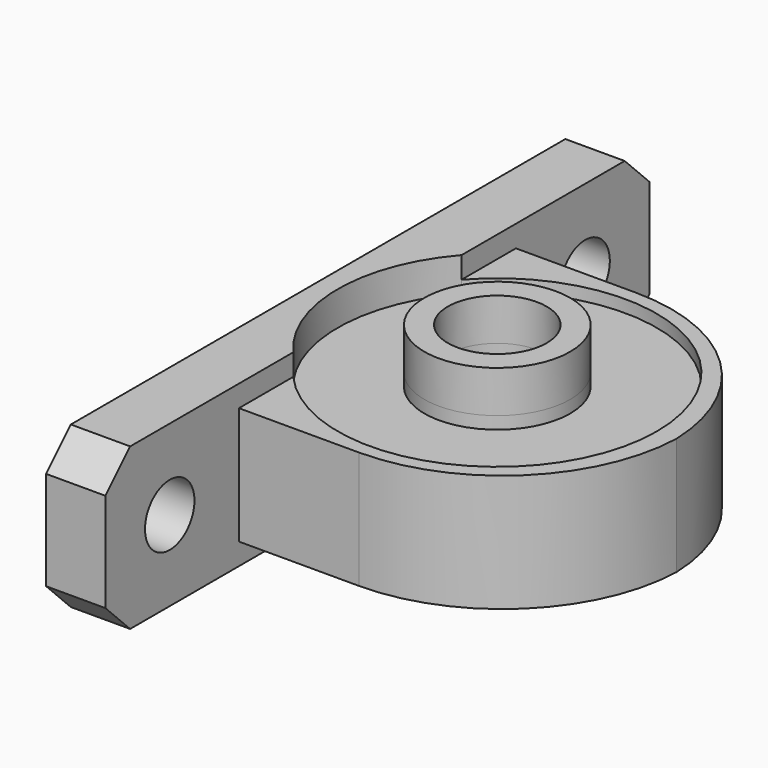
from build123d import *

# Parameters (mm, degrees)
F0_W           = 55
F0_H           = 13
F0_R           = 2.5
F1_DEPTH       = 4.8
F2_DEPTH       = 25
F3_SIZE        = 2.5
F4_W           = 28
F4_H           = 9.5
F5_DEPTH       = 24.2
F6_T1_DEPTH    = 82
F7_R           = 5.9
F8_DEPTH       = 1
F8_DEPTH_BACK  = 25
F9_R           = 4
F10_DEPTH      = 25
F11_R          = 5.9
F12_DEPTH      = 1
F12_DEPTH_BACK = 25
F13_DEPTH      = 9.5
F15_DEPTH      = 1
F9_R_2         = 5.9
F16_DEPTH      = 3.4


# Not quite as in the source:
# - a fillet or chamfer that OpenCascade refuses, or shapes differently, is made with other operations: its cross-section is extruded or revolved along the edge and cut away or added


with BuildPart() as f1:
    # F0 (on Right) → F1 (new body)
    with BuildSketch(Plane.YZ):
        with Locations((27.5, -6.5)):
            Rectangle(F0_W, F0_H)
        with Locations((6.5, -6.5)):
            Circle(F0_R, mode=Mode.SUBTRACT)
        with Locations((48.5, -6.5)):
            Circle(F0_R, mode=Mode.SUBTRACT)
    extrude(amount=F1_DEPTH)

    # F0 (on Right) → F2 (cut)
    with BuildSketch(Plane.YZ):
        with Locations((27.5, -6.5)):
            Rectangle(F0_W, F0_H)
        with Locations((6.5, -6.5)):
            Circle(F0_R, mode=Mode.SUBTRACT)
        with Locations((48.5, -6.5)):
            Circle(F0_R, mode=Mode.SUBTRACT)
    extrude(amount=-F2_DEPTH, mode=Mode.SUBTRACT)

    # F3
    f3_edges = [f1.edges().sort_by_distance(p)[0] for p in [
        (2.4, 0, 0),
        (2.4, 0, -13),
        (2.4, 55, 0),
        (2.4, 55, -13),
    ]]
    chamfer(f3_edges, length=F3_SIZE)

    # F4 (on face) → F5 (join)
    with BuildSketch(Plane.YZ.offset(4.8)):
        with Locations((27.5, -6.5)):
            Rectangle(F4_W, F4_H)
    extrude(amount=F5_DEPTH)

    # F6: fillet of radius 14.5 on 2 edges, made by hand

    # F6_s2 → F6_t1 (cut)
    with BuildSketch(Plane.XY.offset(-47.5)):
        with BuildLine():
            ThreePointArc((14.5, 13.5), (24.753048, 17.746952), (29, 28))
            Line((29, 28), (29, 13.5))
            Line((29, 13.5), (14.5, 13.5))
        make_face()
        with BuildLine():
            ThreePointArc((14.5, 41.5), (24.753048, 37.253048), (29, 27))
            Line((29, 27), (29, 41.5))
            Line((29, 41.5), (14.5, 41.5))
        make_face()
    extrude(amount=F6_T1_DEPTH, mode=Mode.SUBTRACT)

    # F7 (on face) → F8 (cut, two sides)
    with BuildSketch(Plane.XY.offset(-1.75)) as f8_sk:
        with BuildLine():
            ThreePointArc((4.8, 18.990968), (19.041875, 15.427627), (27.395688, 27.5))
            ThreePointArc((27.395688, 27.5), (19.041875, 39.572373), (4.8, 36.009032))
            Line((4.8, 36.009032), (4.8, 18.990968))
        make_face()
        with Locations((14.495688, 27.5)):
            Circle(F7_R, mode=Mode.SUBTRACT)
        with BuildLine():
            Line((4.8, 18.990968), (4.8, 36.009032))
            ThreePointArc((4.8, 36.009032), (1.595688, 27.5), (4.8, 18.990968))
        make_face()
    extrude(amount=-F8_DEPTH, mode=Mode.SUBTRACT)
    extrude(f8_sk.sketch, amount=F8_DEPTH_BACK, mode=Mode.SUBTRACT)

    # F9 (on face) → F10 (cut)
    with BuildSketch(Plane.XY.offset(-1.75)):
        with Locations((14.495688, 27.5)):
            Circle(F9_R)
    extrude(amount=-F10_DEPTH, mode=Mode.SUBTRACT)

    # F11 (on face) → F12 (cut, two sides)
    with BuildSketch(Plane(origin=(0, 0, -11.25), x_dir=(1, 0, 0), z_dir=(0, 0, -1))) as f12_sk:
        with BuildLine():
            ThreePointArc((4.8, -36.009032), (19.041875, -39.572373), (27.395688, -27.5))
            ThreePointArc((27.395688, -27.5), (19.041875, -15.427627), (4.8, -18.990968))
            Line((4.8, -18.990968), (4.8, -36.009032))
        make_face()
        with Locations((14.495688, -27.5)):
            Circle(F11_R, mode=Mode.SUBTRACT)
        with BuildLine():
            Line((4.8, -36.009032), (4.8, -18.990968))
            ThreePointArc((4.8, -18.990968), (1.595688, -27.5), (4.8, -36.009032))
        make_face()
    extrude(amount=-F12_DEPTH, mode=Mode.SUBTRACT)
    extrude(f12_sk.sketch, amount=F12_DEPTH_BACK, mode=Mode.SUBTRACT)


with BuildPart() as f13:
    # F13 (new, through all): a face of the model
    f13_faces = [f1.part.faces().sort_by_distance(p)[0] for p in [
        (8.762566, 27.5, -11.25),
    ]]
    extrude(f13_faces, amount=-F13_DEPTH)


with BuildPart() as f1_1:
    add(f1.part)

    # F14: cut F13
    add(f13.part, mode=Mode.SUBTRACT)


with BuildPart() as f13_1:
    add(f13.part)

    # F15 (cut, through all): a face of the model
    f15_faces = [f13_1.faces().sort_by_distance(p)[0] for p in [
        (8.762566, 27.5, -11.25),
    ]]
    extrude(f15_faces, amount=-F15_DEPTH, mode=Mode.SUBTRACT)

    # F9 (on face) → F16 (join)
    with BuildSketch(Plane.XY.offset(-1.75)):
        with Locations((14.495688, 27.5)):
            Circle(F9_R_2)
        with Locations((14.495688, 27.5)):
            Circle(F9_R, mode=Mode.SUBTRACT)
    extrude(amount=F16_DEPTH)


solid = Compound([f1_1.part, f13_1.part])
